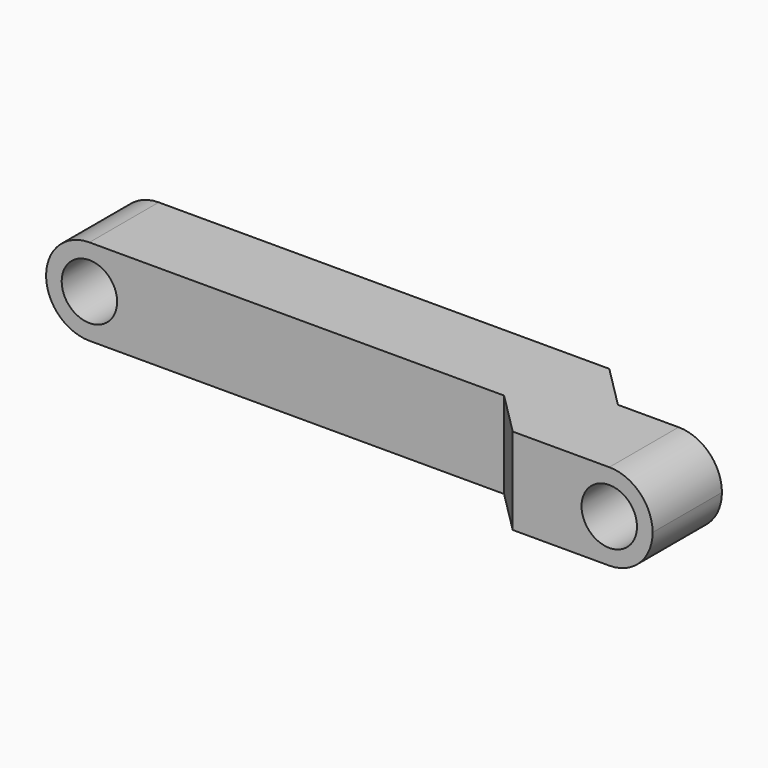
from build123d import *

# Parameters (mm, degrees)
F1_DEPTH = 7.9375
F2_R     = 3.96874
F3_R     = 2.54
F4_DEPTH = 11.90625


# Not quite as in the source:
# - a fillet or chamfer is up to 0.001 mm smaller than in the source, because OpenCascade refuses the exact size


with BuildPart() as f1:
    # F0 (on Top) → F1 (new body)
    with BuildSketch(Plane.XY):
        Polygon((45.24375, 0), (0, 0), (0, -7.9375), (41.9559298487, -7.9375), (45.9246798487, -11.90625), (58.7375, -11.90625), (58.7375, -3.96875), (49.2125, -3.96875), align=None)
    extrude(amount=F1_DEPTH)

    # F2 (radius 3.96875 in the source; OpenCascade refuses exactly that, so slightly less here)
    f2_edges = [f1.edges().sort_by_distance(p)[0] for p in [
        (0, -3.96875, 0),
        (0, -3.96875, 7.9375),
        (58.7375, -7.9375, 0),
        (58.7375, -7.9375, 7.9375),
    ]]
    fillet(f2_edges, radius=F2_R)

    # F3 (on face) → F4 (cut, through all)
    with BuildSketch(Plane(origin=(0, 0, 0), x_dir=(-1, 0, 0), z_dir=(0, 1, 0))):
        with Locations((-3.96875, 3.96875)):
            Circle(F3_R)
        with Locations((-54.76875, 3.96875)):
            Circle(F3_R)
    extrude(amount=-F4_DEPTH, mode=Mode.SUBTRACT)


solid = f1.part
